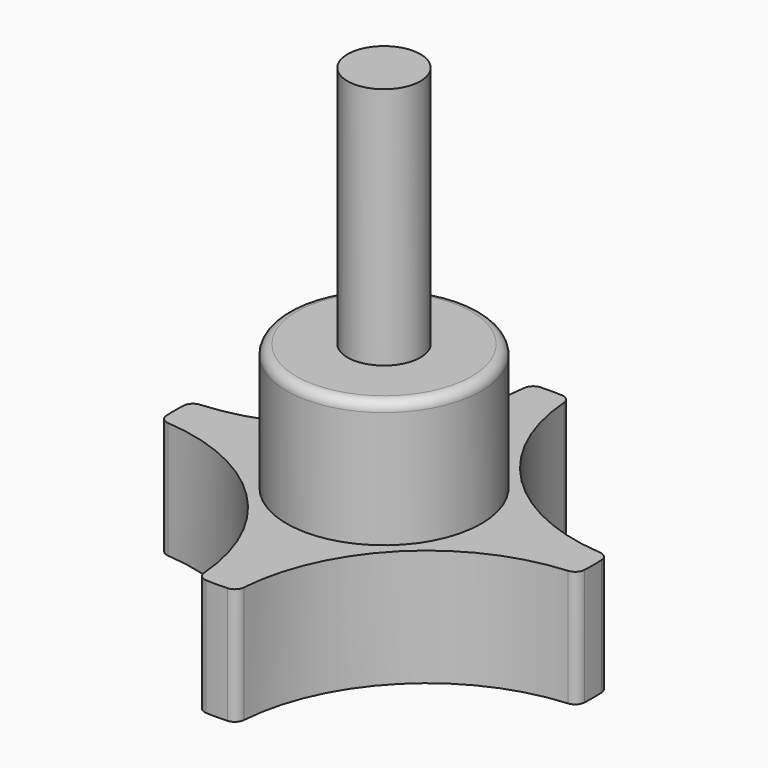
from build123d import *

# Parameters (mm, degrees)
F0_R     = 10
F1_DEPTH = 12
F2_R     = 10
F3_DEPTH = 13
F4_R     = 3.75
F5_DEPTH = 25
F6_R     = 1
F7_R     = 1
F8_DEPTH = 1


with BuildPart() as f1:
    # F0 (on Top) → F1 (new body)
    with BuildSketch(Plane.XY):
        with BuildLine():
            ThreePointArc((-2, 21.4067746286), (-7.8493163593, 7.8493163593), (-21.4067746286, 2))
            ThreePointArc((-21.4067746286, 2), (-21.5, 0), (-21.4067746286, -2))
            ThreePointArc((-21.4067746286, -2), (-7.8493163593, -7.8493163593), (-2, -21.4067746286))
            ThreePointArc((-2, -21.4067746286), (0, -21.5), (2, -21.4067746286))
            ThreePointArc((2, -21.4067746286), (7.8493163593, -7.8493163593), (21.4067746286, -2))
            ThreePointArc((21.4067746286, -2), (21.5, 0), (21.4067746286, 2))
            ThreePointArc((21.4067746286, 2), (7.8493163593, 7.8493163593), (2, 21.4067746286))
            ThreePointArc((2, 21.4067746286), (0, 21.5), (-2, 21.4067746286))
        make_face()
        Circle(F0_R, mode=Mode.SUBTRACT)
        Circle(F0_R)
    extrude(amount=F1_DEPTH)

    # F2 (on face) → F3 (join)
    with BuildSketch(Plane.XY.offset(12)):
        Circle(F2_R)
    extrude(amount=F3_DEPTH)

    # F4 (on face) → F5 (join)
    with BuildSketch(Plane.XY.offset(25)):
        Circle(F4_R)
    extrude(amount=F5_DEPTH)

    # F6
    f6_edges = [f1.edges().sort_by_distance(p)[0] for p in [
        (-10, 0, 25),
    ]]
    fillet(f6_edges, radius=F6_R)

    # F7
    f7_edges = [f1.edges().sort_by_distance(p)[0] for p in [
        (-2, -21.406775, 6),
        (2, -21.406775, 6),
        (-21.406775, -2, 6),
        (-21.406775, 2, 6),
        (-2, 21.406775, 6),
        (2, 21.406775, 6),
        (21.406775, 2, 6),
        (21.406775, -2, 6),
    ]]
    fillet(f7_edges, radius=F7_R)

    # F0 (on Top) → F8 (cut)
    with BuildSketch(Plane.XY):
        Circle(F0_R)
    extrude(amount=F8_DEPTH, mode=Mode.SUBTRACT)


solid = f1.part
